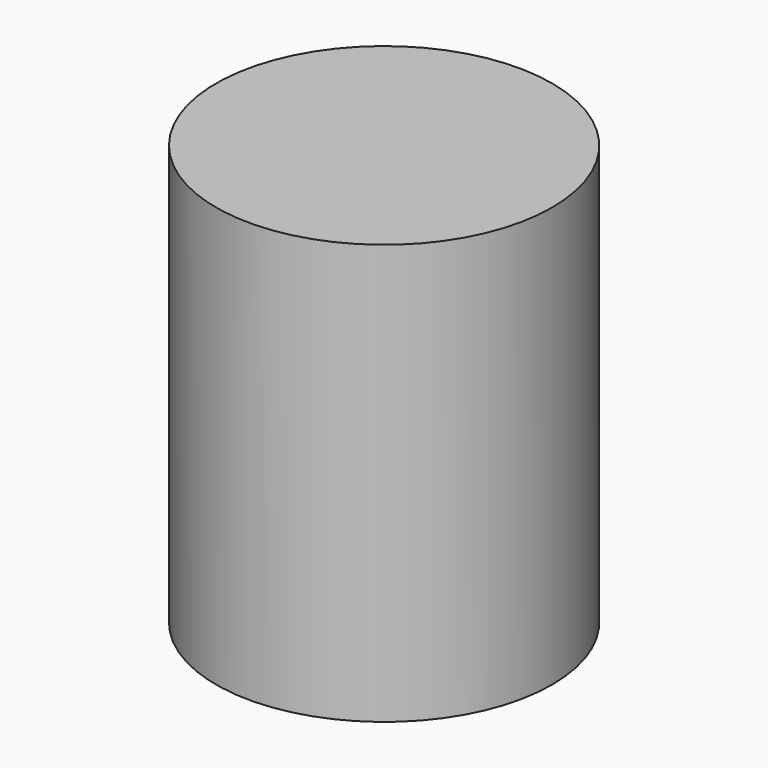
from build123d import *

# Parameters (mm, degrees)
F0_R     = 60
F1_DEPTH = 150
F2_R     = 46
F3_DEPTH = 3


# Not quite as in the source:
# - a feature names something its author has since deleted; it is built from what else it names


with BuildPart() as f1:
    # F0 (on Top) → F1 (new body)
    with BuildSketch(Plane.XY):
        Circle(F0_R)
    extrude(amount=F1_DEPTH)

    # F2 (on face) → F3 (join)
    with BuildSketch(Plane(origin=(0, 0, 0), x_dir=(1, 0, 0), z_dir=(0, 0, -1))):
        Circle(F2_R)
    extrude(amount=F3_DEPTH)

    # F4 (on face) → F5 (revolve, cut)
    with BuildSketch(Plane(origin=(0, 0, -3), x_dir=(1, 0, 0), z_dir=(0, 0, -1))):
        with BuildLine():
            Line((0, 40), (0, -40))
            ThreePointArc((0, -40), (40, 0), (0, 40))
        make_face()
    revolve(axis=Axis((0, 0, -3), (0, -1, 0)), mode=Mode.SUBTRACT)


solid = f1.part
